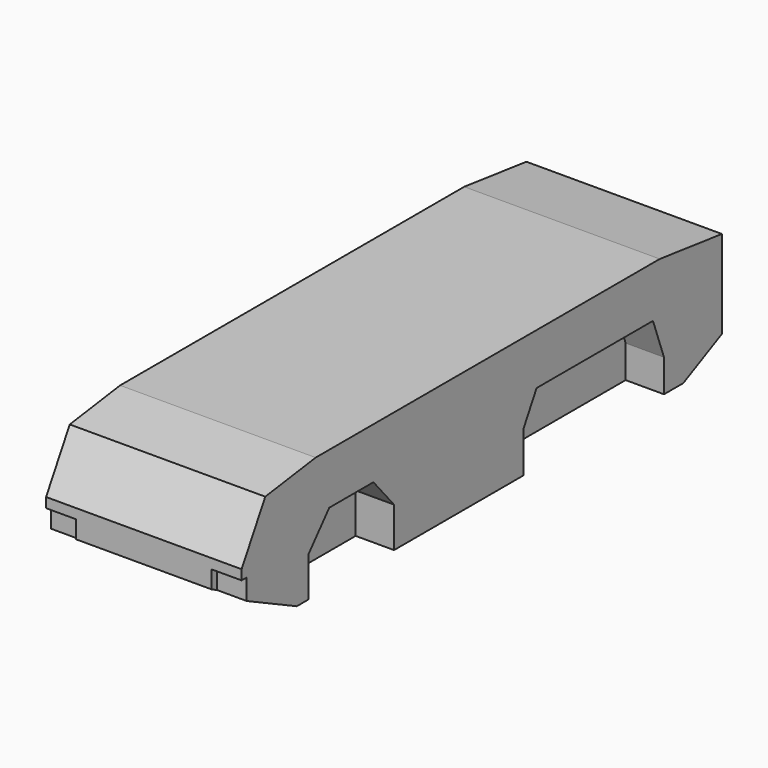
from build123d import *

# Parameters (mm, degrees)
F1_DEPTH = 62.4
F4_DEPTH = 24.5
F5_W     = 19.0535837948
F5_H     = 11.2809054554
F5_H_2   = 2.8878487647
F6_DEPTH = 4.1


# Not quite as in the source:
# - a pattern or mirror of a feature is missing from the dataset's text; its kind, count and spacing are read off the source's solid


with BuildPart() as f1:
    # F0 (on Right) → F1 (new body)
    with BuildSketch(Plane.YZ):
        Polygon((24.6393419802, 87.7444967628), (5.7596671395, 54.6524040401), (5.7596671395, 37.0838306844), (49.7630737395, 15.9439614351), (358.1593094913, 15.9439614351), (388.9961540699, 31.0895591974), (388.9961540699, 87.2576609254), (339.3792808056, 93.3623313904), (64.8232772946, 93.3623313904), align=None)
    extrude(amount=F1_DEPTH)

    # F2: F1 across plane


with BuildPart() as f1_1:
    add(f1.part)
    add(f1.part.mirror(Plane.YZ))

    # F3 (on face) → F4 (cut)
    with BuildSketch(Plane.YZ.offset(62.4)):
        Polygon((59.2419728637, 15.9439614351), (127.3969262838, 15.9439614351), (127.3969262838, 41.5049567819), (110.9381020069, 60.795918107), (75.7007971406, 60.795918107), (59.2419728637, 41.5049567819), align=None)
        Polygon((230.519130826, 15.9439614351), (342.7896499634, 15.9439614351), (342.7896499634, 36.7200672626), (333.9802026749, 60.795918107), (241.1305308342, 60.795918107), (230.519130826, 41.8756008148), align=None)
    f4 = extrude(amount=-F4_DEPTH, mode=Mode.SUBTRACT)

    # F4_copies: F4 across plane
    add(f4.mirror(Plane(origin=(0, 0, 0), x_dir=(0, 0, -1), z_dir=(-1, 0, 0))), mode=Mode.SUBTRACT)

    # F5 (on face) → F6 (cut)
    with BuildSketch(Plane.XZ.offset(-5.7596671395)):
        with Locations((52.8732081026, 42.7242834121)):
            Rectangle(F5_W, F5_H)
        with Locations((52.8732081026, 35.6399063021)):
            Rectangle(F5_W, F5_H_2)
    f6 = extrude(amount=-F6_DEPTH, mode=Mode.SUBTRACT)

    # F6_copies: F6 across plane
    add(f6.mirror(Plane(origin=(0, 0, 0), x_dir=(0, 0, -1), z_dir=(-1, 0, 0))), mode=Mode.SUBTRACT)


solid = f1_1.part
